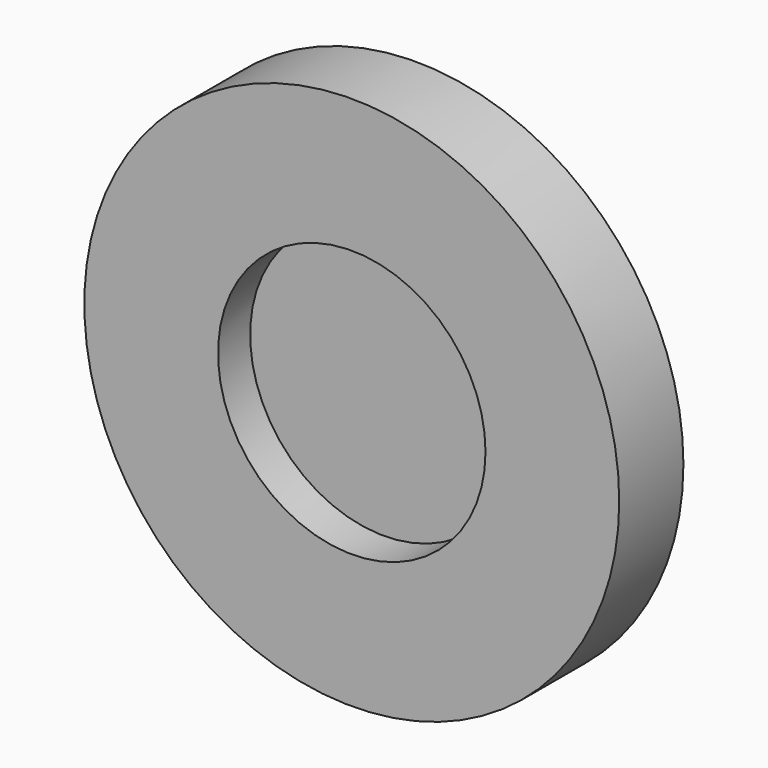
from build123d import *

# Parameters (mm, degrees)
F0_R         = 20
F0_R_2       = 10
F1_DEPTH     = 6
F2_R         = 10
F3_DEPTH     = 3
F4_TEXT_SIZE = 39.2625308135
F5_DEPTH     = 1


# Not quite as in the source:
# - Text() gives the source's letters only with a copy of the font that has no kerning and outlines rounded to 1/6400 em; it was checked with that copy


with BuildPart() as f1:
    # F0 (on Front) → F1 (new body)
    with BuildSketch(Plane.XZ):
        Circle(F0_R)
        Circle(F0_R_2, mode=Mode.SUBTRACT)
        Circle(F0_R_2)
    extrude(amount=F1_DEPTH)

    # F2 (on face) → F3 (cut)
    with BuildSketch(Plane.XZ.offset(6)):
        Circle(F2_R)
    extrude(amount=-F3_DEPTH, mode=Mode.SUBTRACT)

    # F4 (on face) → F5 (join)
    with BuildSketch(Plane(origin=(0, 0, 0), x_dir=(-1, 0, 0), z_dir=(0, 1, 0))):
        with Locations((-14.6783040992, -14.6842001857)):
            Text('G', F4_TEXT_SIZE, font='Open Sans', text_align=(TextAlign.LEFT, TextAlign.BOTTOM))
    extrude(amount=F5_DEPTH)


solid = f1.part
